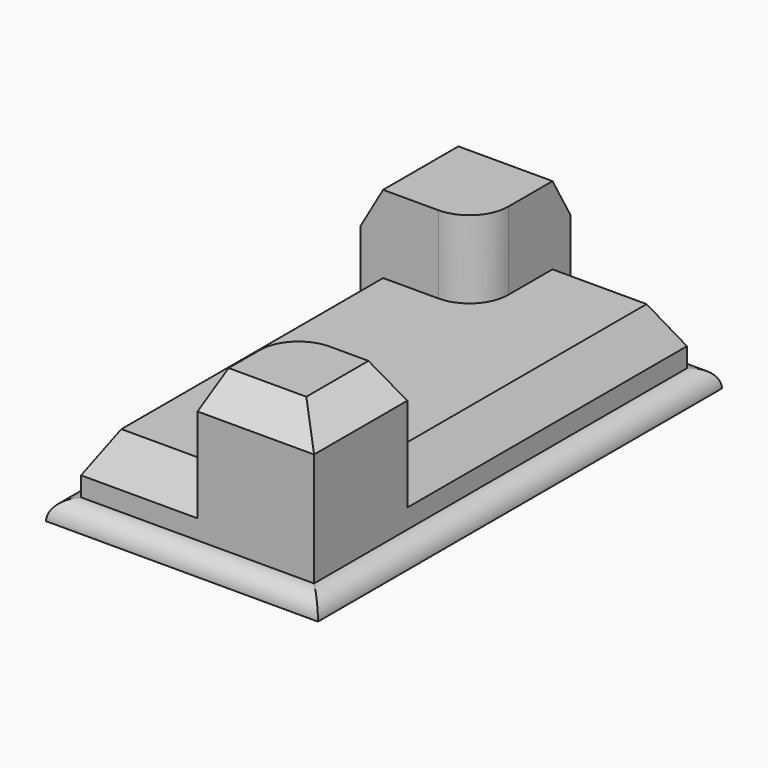
from build123d import *

# Parameters (mm, degrees)
F0_W        = 88.9
F0_H        = 165.1
F1_DEPTH    = 6.35
F2_DEPTH    = 25.4
F3_DEPTH    = 50.8
F4_C1_SIZE2 = 7.3323484187
F4_C1_SIZE  = 12.7
F4_C2_SIZE2 = 7.3323484187
F4_C2_SIZE  = 12.7
F4_C3_SIZE2 = 12.7
F4_C3_SIZE  = 7.3323484187
F4_C4_SIZE2 = 12.7
F4_C4_SIZE  = 7.3323484187
F5_R        = 6.34999
F6_C1_SIZE2 = 7.3323484187
F6_C1_SIZE  = 12.7
F6_C2_SIZE2 = 7.3323484187
F6_C2_SIZE  = 12.7
F6_C3_SIZE2 = 12.7
F6_C3_SIZE  = 7.3323484187
F6_C4_SIZE2 = 12.7
F6_C4_SIZE  = 7.3323484187


# Not quite as in the source:
# - a fillet or chamfer is up to 0.001 mm smaller than in the source, because OpenCascade refuses the exact size


with BuildPart() as f1:
    # F0 (on Top) → F1 (new body)
    with BuildSketch(Plane.XY):
        Rectangle(F0_W, F0_H)
        Polygon((0, 76.2), (38.1, 76.2), (38.1, -38.1), (38.1, -76.2), (0, -76.2), (-38.1, -76.2), (-38.1, 38.1), (-38.1, 76.2), align=None, mode=Mode.SUBTRACT)
        with BuildLine():
            Line((0, 50.8), (0, 76.2))
            Line((0, 76.2), (-38.1, 76.2))
            Line((-38.1, 76.2), (-38.1, 38.1))
            Line((-38.1, 38.1), (-12.7, 38.1))
            ThreePointArc((-12.7, 38.1), (-3.7197438789, 41.8197438789), (0, 50.8))
        make_face()
        with BuildLine():
            Line((38.1, -38.1), (38.1, 76.2))
            Line((38.1, 76.2), (0, 76.2))
            Line((0, 76.2), (0, 50.8))
            ThreePointArc((0, 50.8), (-3.7197438789, 41.8197438789), (-12.7, 38.1))
            Line((-12.7, 38.1), (-38.1, 38.1))
            Line((-38.1, 38.1), (-38.1, -76.2))
            Line((-38.1, -76.2), (0, -76.2))
            Line((0, -76.2), (0, -50.8))
            ThreePointArc((0, -50.8), (3.7197438789, -41.8197438789), (12.7, -38.1))
            Line((12.7, -38.1), (38.1, -38.1))
        make_face()
        with BuildLine():
            Line((38.1, -76.2), (38.1, -38.1))
            Line((38.1, -38.1), (12.7, -38.1))
            ThreePointArc((12.7, -38.1), (3.7197438789, -41.8197438789), (0, -50.8))
            Line((0, -50.8), (0, -76.2))
            Line((0, -76.2), (38.1, -76.2))
        make_face()
    extrude(amount=F1_DEPTH)

    # F0 (on Top) → F2 (join)
    with BuildSketch(Plane.XY):
        with BuildLine():
            Line((38.1, -38.1), (38.1, 76.2))
            Line((38.1, 76.2), (0, 76.2))
            Line((0, 76.2), (0, 50.8))
            ThreePointArc((0, 50.8), (-3.7197438789, 41.8197438789), (-12.7, 38.1))
            Line((-12.7, 38.1), (-38.1, 38.1))
            Line((-38.1, 38.1), (-38.1, -76.2))
            Line((-38.1, -76.2), (0, -76.2))
            Line((0, -76.2), (0, -50.8))
            ThreePointArc((0, -50.8), (3.7197438789, -41.8197438789), (12.7, -38.1))
            Line((12.7, -38.1), (38.1, -38.1))
        make_face()
        with BuildLine():
            Line((0, 50.8), (0, 76.2))
            Line((0, 76.2), (-38.1, 76.2))
            Line((-38.1, 76.2), (-38.1, 38.1))
            Line((-38.1, 38.1), (-12.7, 38.1))
            ThreePointArc((-12.7, 38.1), (-3.7197438789, 41.8197438789), (0, 50.8))
        make_face()
        with BuildLine():
            Line((38.1, -76.2), (38.1, -38.1))
            Line((38.1, -38.1), (12.7, -38.1))
            ThreePointArc((12.7, -38.1), (3.7197438789, -41.8197438789), (0, -50.8))
            Line((0, -50.8), (0, -76.2))
            Line((0, -76.2), (38.1, -76.2))
        make_face()
    extrude(amount=F2_DEPTH)

    # F0 (on Top) → F3 (join)
    with BuildSketch(Plane.XY):
        with BuildLine():
            Line((0, 50.8), (0, 76.2))
            Line((0, 76.2), (-38.1, 76.2))
            Line((-38.1, 76.2), (-38.1, 38.1))
            Line((-38.1, 38.1), (-12.7, 38.1))
            ThreePointArc((-12.7, 38.1), (-3.7197438789, 41.8197438789), (0, 50.8))
        make_face()
        with BuildLine():
            Line((38.1, -76.2), (38.1, -38.1))
            Line((38.1, -38.1), (12.7, -38.1))
            ThreePointArc((12.7, -38.1), (3.7197438789, -41.8197438789), (0, -50.8))
            Line((0, -50.8), (0, -76.2))
            Line((0, -76.2), (38.1, -76.2))
        make_face()
    extrude(amount=F3_DEPTH)

    # F4: chamfer of 12.7 x 7.3323484187 on 4 edges, made by hand

    # F4_c1
    f4_c1_edges = [f1.edges().sort_by_distance(p)[0] for p in [
        (-19.05, -76.2, 25.4),
    ]]
    f4_c1_side = f1.faces().sort_by_distance((-19.05, -76.2, 25.2533530316))[0]
    chamfer(f4_c1_edges, length=F4_C1_SIZE, length2=F4_C1_SIZE2, reference=f4_c1_side)

    # F4_c2
    f4_c2_edges = [f1.edges().sort_by_distance(p)[0] for p in [
        (38.1, 19.05, 25.4),
    ]]
    f4_c2_side = f1.faces().sort_by_distance((38.1, 19.05, 25.2533530316))[0]
    chamfer(f4_c2_edges, length=F4_C2_SIZE, length2=F4_C2_SIZE2, reference=f4_c2_side)

    # F4_c3
    f4_c3_edges = [f1.edges().sort_by_distance(p)[0] for p in [
        (-38.1, -15.3838257906, 25.4),
    ]]
    f4_c3_side = f1.faces().sort_by_distance((-37.9533530316, -15.3838257906, 25.4))[0]
    chamfer(f4_c3_edges, length=F4_C3_SIZE, length2=F4_C3_SIZE2, reference=f4_c3_side)

    # F4_c4
    f4_c4_edges = [f1.edges().sort_by_distance(p)[0] for p in [
        (15.3838257906, 76.2, 25.4),
    ]]
    f4_c4_side = f1.faces().sort_by_distance((15.3838257906, 76.0533530316, 25.4))[0]
    chamfer(f4_c4_edges, length=F4_C4_SIZE, length2=F4_C4_SIZE2, reference=f4_c4_side)

    # F5 (radius 6.35 in the source; OpenCascade refuses exactly that, so slightly less here)
    f5_edges = [f1.edges().sort_by_distance(p)[0] for p in [
        (0, 82.55, 6.35),
        (44.45, 0, 6.35),
        (-44.45, 0, 6.35),
        (0, -82.55, 6.35),
    ]]
    fillet(f5_edges, radius=F5_R)

    # F6: chamfer of 12.7 x 7.3323484187 on 4 edges, made by hand

    # F6_c1
    f6_c1_edges = [f1.edges().sort_by_distance(p)[0] for p in [
        (-38.1, 57.15, 50.8),
    ]]
    f6_c1_side = f1.faces().sort_by_distance((-38.1, 57.15, 50.6533530316))[0]
    chamfer(f6_c1_edges, length=F6_C1_SIZE, length2=F6_C1_SIZE2, reference=f6_c1_side)

    # F6_c2
    f6_c2_edges = [f1.edges().sort_by_distance(p)[0] for p in [
        (-15.3838257906, 76.2, 50.8),
    ]]
    f6_c2_side = f1.faces().sort_by_distance((-15.3838257906, 76.2, 50.6533530316))[0]
    chamfer(f6_c2_edges, length=F6_C2_SIZE, length2=F6_C2_SIZE2, reference=f6_c2_side)

    # F6_c3
    f6_c3_edges = [f1.edges().sort_by_distance(p)[0] for p in [
        (38.1, -57.15, 50.8),
    ]]
    f6_c3_side = f1.faces().sort_by_distance((38.1, -57.15, 50.6533530316))[0]
    chamfer(f6_c3_edges, length=F6_C3_SIZE, length2=F6_C3_SIZE2, reference=f6_c3_side)

    # F6_c4
    f6_c4_edges = [f1.edges().sort_by_distance(p)[0] for p in [
        (12.7, -76.2, 50.8),
    ]]
    f6_c4_side = f1.faces().sort_by_distance((12.7, -76.2, 50.6533530316))[0]
    chamfer(f6_c4_edges, length=F6_C4_SIZE, length2=F6_C4_SIZE2, reference=f6_c4_side)


solid = f1.part
